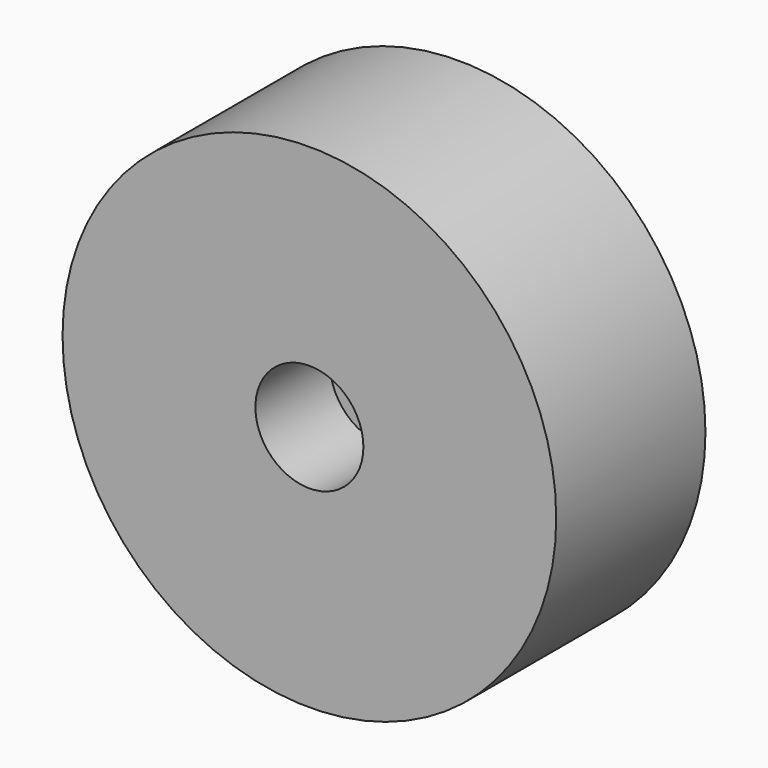
from build123d import *

# Parameters (mm, degrees)
F0_R     = 33.613844165
F0_R_2   = 7.3530240303
F1_DEPTH = 12.7
F2_DEPTH = 25.4


with BuildPart() as f1:
    # F0 (on Front) → F1 (new body)
    with BuildSketch(Plane.XZ):
        Circle(F0_R)
        with BuildLine():
            ThreePointArc((4.7208512746, -19.951569966), (4.6925332266, -19.9590350044), (4.6642082743, -19.9664738029))
            ThreePointArc((4.6642082743, -19.9664738029), (4.6934800842, -19.9547063806), (4.7227373879, -19.9429029377))
            ThreePointArc((4.7227373879, -19.9429029377), (4.7217944882, -19.947236486), (4.7208512746, -19.951569966))
        make_face(mode=Mode.SUBTRACT)
        Circle(F0_R_2, mode=Mode.SUBTRACT)
        with BuildLine():
            ThreePointArc((14.5159144375, 14.0511614861), (14.5316083012, 14.029833317), (14.547274448, 14.0084847808))
            ThreePointArc((14.547274448, 14.0084847808), (14.5285756501, 14.0288524457), (14.5098472673, 14.0491929102))
            ThreePointArc((14.5098472673, 14.0491929102), (14.5128808291, 14.0501772698), (14.5159144375, 14.0511614861))
        make_face(mode=Mode.SUBTRACT)
        Circle(F0_R_2)
    extrude(amount=F1_DEPTH)

    # F0 (on Front) → F2 (join)
    with BuildSketch(Plane.XZ):
        Circle(F0_R)
        with BuildLine():
            ThreePointArc((4.7208512746, -19.951569966), (4.6925332266, -19.9590350044), (4.6642082743, -19.9664738029))
            ThreePointArc((4.6642082743, -19.9664738029), (4.6934800842, -19.9547063806), (4.7227373879, -19.9429029377))
            ThreePointArc((4.7227373879, -19.9429029377), (4.7217944882, -19.947236486), (4.7208512746, -19.951569966))
        make_face(mode=Mode.SUBTRACT)
        Circle(F0_R_2, mode=Mode.SUBTRACT)
        with BuildLine():
            ThreePointArc((14.5159144375, 14.0511614861), (14.5316083012, 14.029833317), (14.547274448, 14.0084847808))
            ThreePointArc((14.547274448, 14.0084847808), (14.5285756501, 14.0288524457), (14.5098472673, 14.0491929102))
            ThreePointArc((14.5098472673, 14.0491929102), (14.5128808291, 14.0501772698), (14.5159144375, 14.0511614861))
        make_face(mode=Mode.SUBTRACT)
    extrude(amount=F2_DEPTH)


solid = f1.part
